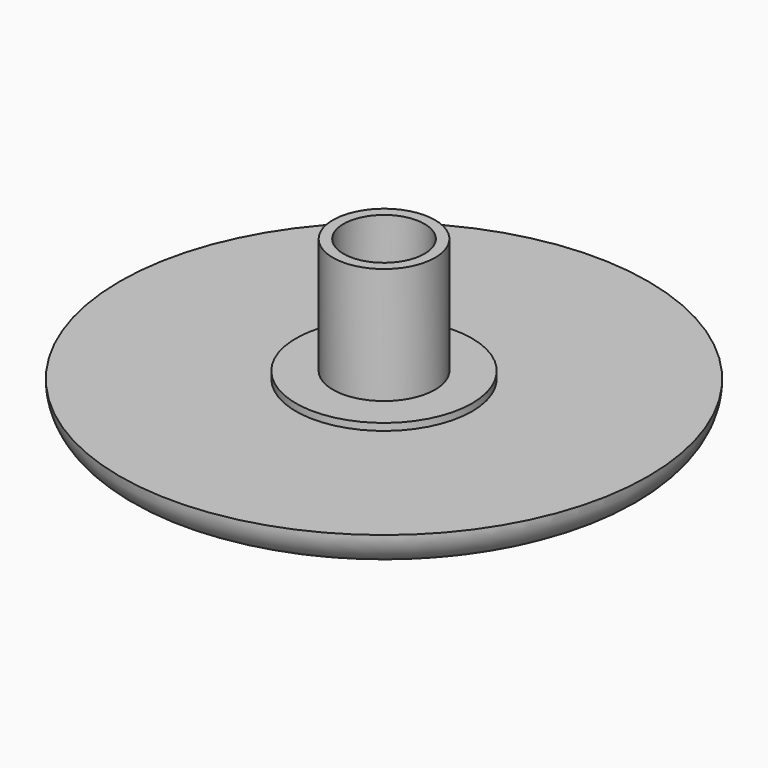
from build123d import *

# Parameters (mm, degrees)
F0_R     = 2.9
F1_DEPTH = 7
F2_T     = -0.6
F0_R_2   = 15
F0_R_3   = 5
F3_DEPTH = 2
F4_R     = 1.99999
F7_R     = 0.3
F8_DEPTH = 0.4


# Not quite as in the source:
# - a fillet or chamfer is up to 0.001 mm smaller than in the source, because OpenCascade refuses the exact size


with BuildPart() as f1:
    # F0 (on Top) → F1 (new body)
    with BuildSketch(Plane.XY):
        Circle(F0_R)
    extrude(amount=F1_DEPTH)

    # F2
    f2_openings = [f1.faces().sort_by_distance(p)[0] for p in [
        (0, 0, 7),
    ]]
    offset(amount=F2_T, openings=f2_openings)

    # F0 (on Top) → F3 (join)
    with BuildSketch(Plane.XY):
        Circle(F0_R_2)
        Circle(F0_R_3, mode=Mode.SUBTRACT)
        Circle(F0_R_3)
        Circle(F0_R, mode=Mode.SUBTRACT)
        Circle(F0_R)
    extrude(amount=-F3_DEPTH)

    # F4 (radius 2 in the source; OpenCascade refuses exactly that, so slightly less here)
    f4_edges = [f1.edges().sort_by_distance(p)[0] for p in [
        (-15, 0, -2),
    ]]
    fillet(f4_edges, radius=F4_R)

    # F5 (on Front) → F6 (revolve, cut)
    with BuildSketch(Plane.XZ):
        with BuildLine():
            ThreePointArc((2.175, 3.5), (2.2116116524, 3.4116116524), (2.3, 3.375))
            Line((2.3, 3.375), (2.3, 3.5))
            Line((2.3, 3.5), (2.175, 3.5))
        make_face()
        with BuildLine():
            Line((2.3, 3.5), (2.3, 3.375))
            ThreePointArc((2.3, 3.375), (2.3883883476, 3.4116116524), (2.425, 3.5))
            ThreePointArc((2.425, 3.5), (2.3, 3.625), (2.175, 3.5))
            Line((2.175, 3.5), (2.3, 3.5))
        make_face()
    revolve(axis=Axis((0, 0, 1.75), (0, 0, 1)), mode=Mode.SUBTRACT)

    # F7
    f7_edges = [f1.edges().sort_by_distance(p)[0] for p in [
        (-2.3, 0, 3.375),
    ]]
    fillet(f7_edges, radius=F7_R)

    # F0 (on Top) → F8 (join)
    with BuildSketch(Plane.XY):
        Circle(F0_R_3)
        Circle(F0_R, mode=Mode.SUBTRACT)
    extrude(amount=F8_DEPTH)


solid = f1.part
